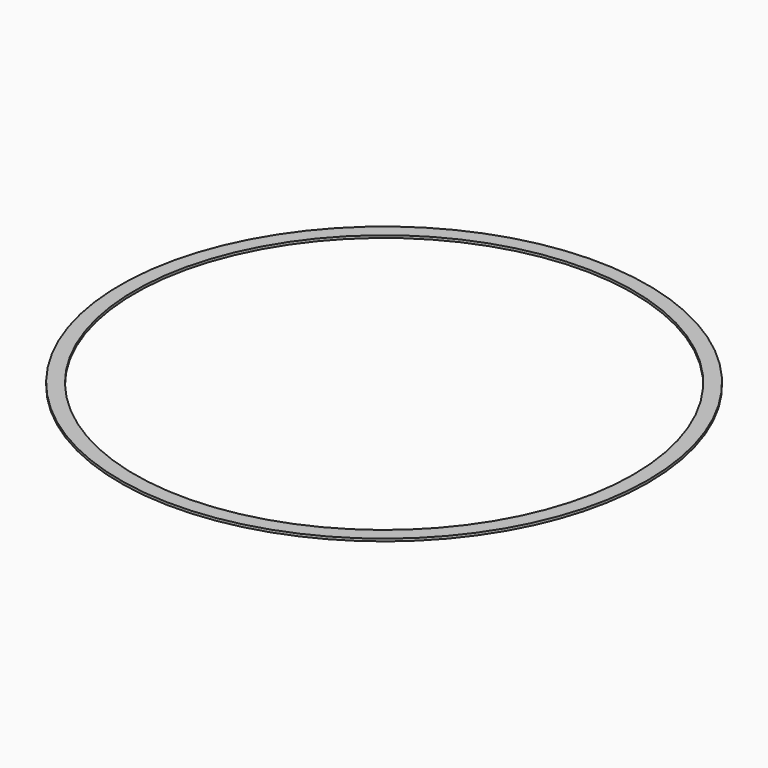
from build123d import *

# Parameters (mm, degrees)
F0_R     = 455.54138
F0_R_2   = 430.14138
F1_DEPTH = 4.2333333333


# Not quite as in the source:
# - a length typed as a fraction of an inch, garbled in the dataset ("3 / 203.2 mm" for 3/8 in), is restored


with BuildPart() as f1:
    # F0 (on Top) → F1 (new body)
    with BuildSketch(Plane.XY):
        Circle(F0_R)
        Circle(F0_R_2, mode=Mode.SUBTRACT)
    extrude(amount=F1_DEPTH)


solid = f1.part
